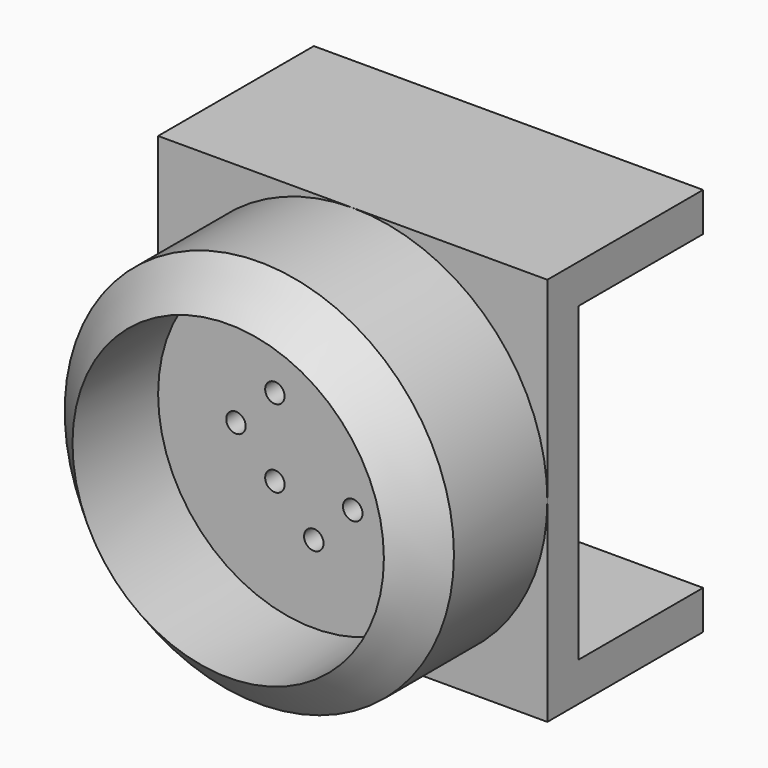
from build123d import *

# Parameters (mm, degrees)
F0_R     = 12.7
F0_R_2   = 10.16
F1_DEPTH = 12.7
F0_R_3   = 0.635
F2_DEPTH = 3.175
F4_DEPTH = 12.7
F3_R     = 0.635
F5_DEPTH = 2.54


# Not quite as in the source:
# - a fillet or chamfer that OpenCascade refuses, or shapes differently, is made with other operations: its cross-section is extruded or revolved along the edge and cut away or added


with BuildPart() as f1:
    # F0 (on Front) → F1 (new body)
    with BuildSketch(Plane.XZ):
        Circle(F0_R)
        Circle(F0_R_2, mode=Mode.SUBTRACT)
    extrude(amount=F1_DEPTH)

    # F0 (on Front) → F2 (join)
    with BuildSketch(Plane.XZ):
        Circle(F0_R_2)
        with Locations((0, -5.08)):
            Circle(F0_R_3, mode=Mode.SUBTRACT)
        with Locations((-5.08, 0)):
            Circle(F0_R_3, mode=Mode.SUBTRACT)
        with Locations((-2.54, -2.54)):
            Circle(F0_R_3, mode=Mode.SUBTRACT)
        with Locations((2.54, -2.54)):
            Circle(F0_R_3, mode=Mode.SUBTRACT)
        with Locations((5.08, 0)):
            Circle(F0_R_3, mode=Mode.SUBTRACT)
        with Locations((-2.54, 2.54)):
            Circle(F0_R_3, mode=Mode.SUBTRACT)
        with Locations((0, 5.08)):
            Circle(F0_R_3, mode=Mode.SUBTRACT)
        with Locations((2.54, 2.54)):
            Circle(F0_R_3, mode=Mode.SUBTRACT)
    extrude(amount=F2_DEPTH)

    # F3 (on face) → F4 (join)
    with BuildSketch(Plane(origin=(0, 0, 0), x_dir=(-1, 0, 0), z_dir=(0, 1, 0))):
        with BuildLine():
            ThreePointArc((-7.62, 10.16), (-4.0160926196, 12.0482778882), (1.86e-08, 12.7))
            Line((1.86e-08, 12.7), (-12.7, 12.7))
            Line((-12.7, 12.7), (-12.7, 10.16))
            Line((-12.7, 10.16), (-7.62, 10.16))
        make_face()
        with BuildLine():
            ThreePointArc((7.62, 10.16), (4.0160926372, 12.0482778823), (1.86e-08, 12.7))
            ThreePointArc((1.86e-08, 12.7), (-4.0160926196, 12.0482778882), (-7.62, 10.16))
            Line((-7.62, 10.16), (7.62, 10.16))
        make_face()
        with BuildLine():
            Line((12.7, 10.16), (12.7, 12.7))
            Line((12.7, 12.7), (1.86e-08, 12.7))
            ThreePointArc((1.86e-08, 12.7), (4.0160926372, 12.0482778823), (7.62, 10.16))
            Line((7.62, 10.16), (12.7, 10.16))
        make_face()
        with BuildLine():
            Line((12.7, -12.7), (12.7, -10.16))
            Line((12.7, -10.16), (7.62, -10.16))
            ThreePointArc((7.62, -10.16), (4.0160926284, -12.0482778852), (0, -12.7))
            Line((0, -12.7), (12.7, -12.7))
        make_face()
        with BuildLine():
            ThreePointArc((0, -12.7), (4.0160926284, -12.0482778852), (7.62, -10.16))
            Line((7.62, -10.16), (-7.62, -10.16))
            ThreePointArc((-7.62, -10.16), (-4.0160926284, -12.0482778852), (0, -12.7))
        make_face()
        with BuildLine():
            Line((-7.62, -10.16), (-12.7, -10.16))
            Line((-12.7, -10.16), (-12.7, -12.7))
            Line((-12.7, -12.7), (0, -12.7))
            ThreePointArc((0, -12.7), (-4.0160926284, -12.0482778852), (-7.62, -10.16))
        make_face()
    extrude(amount=F4_DEPTH)

    # F3 (on face) → F5 (join)
    with BuildSketch(Plane(origin=(0, 0, 0), x_dir=(-1, 0, 0), z_dir=(0, 1, 0))):
        with BuildLine():
            Line((12.7, 0), (12.7, 10.16))
            Line((12.7, 10.16), (7.62, 10.16))
            ThreePointArc((7.62, 10.16), (11.3592253257, 5.6796126628), (12.7, 0))
        make_face()
        with BuildLine():
            ThreePointArc((12.7, 0), (11.3592253257, 5.6796126628), (7.62, 10.16))
            Line((7.62, 10.16), (-7.62, 10.16))
            ThreePointArc((-7.62, 10.16), (-11.3592253257, 5.6796126628), (-12.7, 0))
            ThreePointArc((-12.7, 0), (-11.3592253257, -5.6796126628), (-7.62, -10.16))
            Line((-7.62, -10.16), (7.62, -10.16))
            ThreePointArc((7.62, -10.16), (11.3592253257, -5.6796126628), (12.7, 0))
        make_face()
        with Locations((0, -5.08)):
            Circle(F3_R, mode=Mode.SUBTRACT)
        with Locations((-5.08, 0)):
            Circle(F3_R, mode=Mode.SUBTRACT)
        with Locations((-2.54, -2.54)):
            Circle(F3_R, mode=Mode.SUBTRACT)
        with Locations((2.54, -2.54)):
            Circle(F3_R, mode=Mode.SUBTRACT)
        with Locations((5.08, 0)):
            Circle(F3_R, mode=Mode.SUBTRACT)
        with Locations((-2.54, 2.54)):
            Circle(F3_R, mode=Mode.SUBTRACT)
        with Locations((0, 5.08)):
            Circle(F3_R, mode=Mode.SUBTRACT)
        with Locations((2.54, 2.54)):
            Circle(F3_R, mode=Mode.SUBTRACT)
        with BuildLine():
            ThreePointArc((-12.7, 0), (-11.3592253257, 5.6796126628), (-7.62, 10.16))
            Line((-7.62, 10.16), (-12.7, 10.16))
            Line((-12.7, 10.16), (-12.7, 0))
        make_face()
        with BuildLine():
            Line((12.7, -10.16), (12.7, 0))
            ThreePointArc((12.7, 0), (11.3592253257, -5.6796126628), (7.62, -10.16))
            Line((7.62, -10.16), (12.7, -10.16))
        make_face()
        with BuildLine():
            ThreePointArc((-7.62, -10.16), (-11.3592253257, -5.6796126628), (-12.7, 0))
            Line((-12.7, 0), (-12.7, -10.16))
            Line((-12.7, -10.16), (-7.62, -10.16))
        make_face()
    extrude(amount=F5_DEPTH)

    # F6: chamfer of 5.08 on 1 edges, made by hand

    # F6_s1 → F6_t2 (revolve, cut)
    with BuildSketch(Plane.XY):
        Polygon((12.7, -7.62), (7.62, -12.7), (12.7, -12.7), align=None)
    revolve(axis=Axis((0, -12.7, 0), (0, -1, 0)), mode=Mode.SUBTRACT)


solid = f1.part
